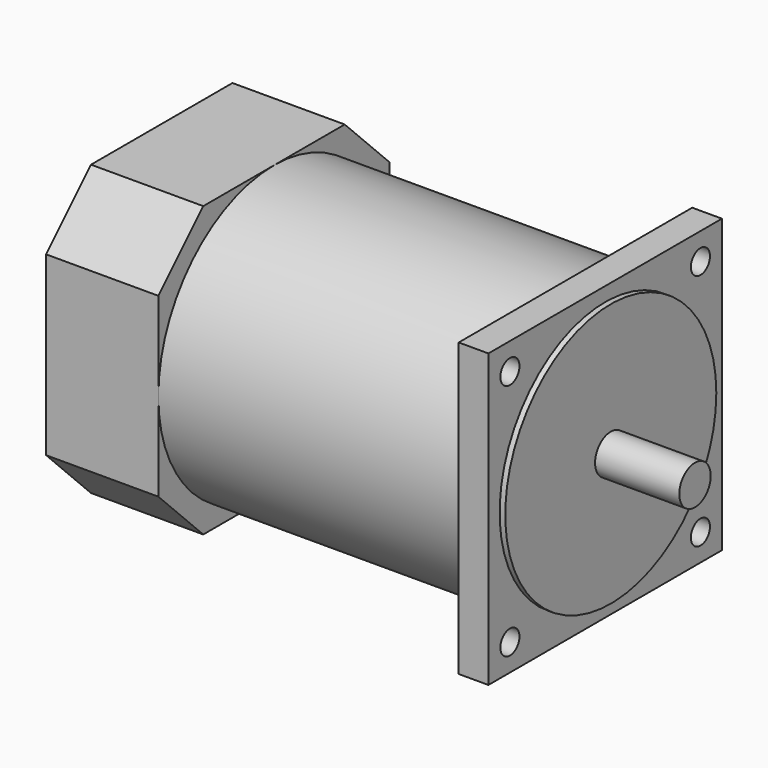
from build123d import *

# Parameters (mm, degrees)
F0_W      = 104
F0_H      = 104
F1_DEPTH  = 160
F3_W      = 107.42
F3_H      = 40
F5_W      = 104
F5_H      = 104
F5_W_2    = 103
F5_H_2    = 103
F6_DEPTH  = 40
F7_SIZE   = 20
F8_R      = 4.25
F9_DEPTH  = 25
F10_R     = 7
F11_DEPTH = 30
F12_W     = 104
F12_H     = 104
F12_R     = 4.25
F12_R_2   = 47
F13_DEPTH = 2


with BuildPart() as f1:
    # F0 (on Right) → F1 (new body)
    with BuildSketch(Plane.YZ):
        with Locations((52, 52)):
            Rectangle(F0_W, F0_H)
    extrude(amount=-F1_DEPTH)

    # F3 (on offset) → F4 (revolve, cut)
    with BuildSketch(Plane.XZ.offset(-52)):
        with Locations((-66.29, 123.5)):
            Rectangle(F3_W, F3_H)
    revolve(axis=Axis((-69.2846309394, 52, 52), (1, 0, 0)), mode=Mode.SUBTRACT)

    # F5 (on face) → F6 (cut)
    with BuildSketch(Plane(origin=(-160, 0, 0), x_dir=(0, -1, 0), z_dir=(-1, 0, 0))):
        with Locations((-52, 52)):
            Rectangle(F5_W, F5_H)
        with Locations((-52, 52)):
            Rectangle(F5_W_2, F5_H_2, mode=Mode.SUBTRACT)
    extrude(amount=-F6_DEPTH, mode=Mode.SUBTRACT)

    # F7
    f7_edges = [f1.edges().sort_by_distance(p)[0] for p in [
        (-140, 0.5, 103.5),
        (-140, 103.5, 103.5),
        (-140, 103.5, 0.5),
        (-140, 0.5, 0.5),
    ]]
    chamfer(f7_edges, length=F7_SIZE)

    # F8 (on face) → F9 (cut)
    with BuildSketch(Plane.YZ):
        with Locations((94.4264068712, 94.4264068712)):
            Circle(F8_R)
        with Locations((94.4264068712, 9.5735931288)):
            Circle(F8_R)
        with Locations((9.5735931288, 94.4264068712)):
            Circle(F8_R)
        with Locations((9.5735931288, 9.5735931288)):
            Circle(F8_R)
    extrude(amount=-F9_DEPTH, mode=Mode.SUBTRACT)

    # F10 (on face) → F11 (join)
    with BuildSketch(Plane.YZ):
        with Locations((52, 52)):
            Circle(F10_R)
    extrude(amount=F11_DEPTH)

    # F12 (on face) → F13 (cut)
    with BuildSketch(Plane.YZ):
        with Locations((52, 52)):
            Rectangle(F12_W, F12_H)
        with Locations((9.5735931288, 9.5735931288)):
            Circle(F12_R, mode=Mode.SUBTRACT)
        with Locations((94.4264068712, 9.5735931288)):
            Circle(F12_R, mode=Mode.SUBTRACT)
        with Locations((9.5735931288, 94.4264068712)):
            Circle(F12_R, mode=Mode.SUBTRACT)
        with Locations((52, 52)):
            Circle(F12_R_2, mode=Mode.SUBTRACT)
        with Locations((94.4264068712, 94.4264068712)):
            Circle(F12_R, mode=Mode.SUBTRACT)
    extrude(amount=-F13_DEPTH, mode=Mode.SUBTRACT)


solid = f1.part
